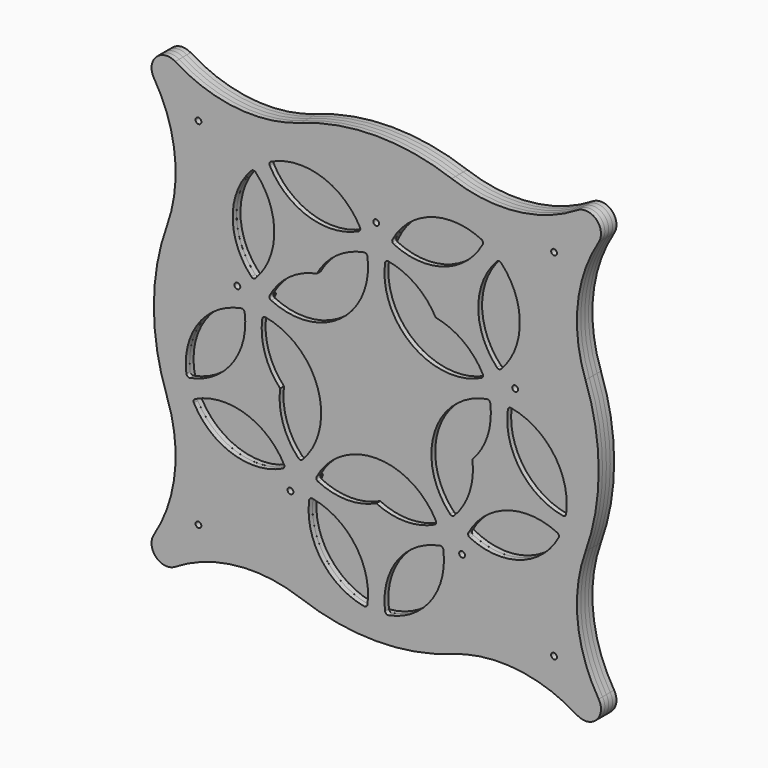
from build123d import *

# Parameters (mm, degrees)
F2_DEPTH  = 2.5
F4_DEPTH  = 2.5
F6_DEPTH  = 2.5
F8_DEPTH  = 2.5
F9_R      = 1.5
F10_DEPTH = 25
F11_DEPTH = 355


# Not quite as in the source:
# - an extrude ends at something that could not be found from the text; its depth is read off the source's solid


with BuildPart() as f2:
    # F1 (on Front) → F2 (new body)
    with BuildSketch(Plane.XZ):
        with BuildLine():
            ThreePointArc((24.0259388064, -87.5519624316), (57.2853373786, -83.5126697988), (88.9850116486, -94.3585966628))
            ThreePointArc((88.9850116486, -94.3585966628), (98.8568675438, -93.2159096685), (99.9995545382, -83.3440537732))
            ThreePointArc((99.9995545382, -83.3440537732), (89.1536276742, -51.6443795033), (93.192920307, -18.384980931))
            ThreePointArc((93.192920307, -18.384980931), (100.0126757728, 20.6282821025), (93.192920307, 59.6415451361))
            ThreePointArc((93.192920307, 59.6415451361), (89.1536276742, 92.9009437083), (99.9995545382, 124.6006179783))
            ThreePointArc((99.9995545382, 124.6006179783), (98.8568675438, 134.4724738736), (88.9850116486, 135.6151608679))
            ThreePointArc((88.9850116486, 135.6151608679), (57.2853373786, 124.7692340039), (24.0259388064, 128.8085266367))
            ThreePointArc((24.0259388064, 128.8085266367), (-14.9873242272, 135.6282821025), (-54.0005872607, 128.8085266367))
            ThreePointArc((-54.0005872607, 128.8085266367), (-87.259985833, 124.7692340039), (-118.959660103, 135.6151608679))
            ThreePointArc((-118.959660103, 135.6151608679), (-128.8315159982, 134.4724738736), (-129.9742029925, 124.6006179783))
            ThreePointArc((-129.9742029925, 124.6006179783), (-119.1282761286, 92.9009437083), (-123.1675687614, 59.6415451361))
            ThreePointArc((-123.1675687614, 59.6415451361), (-129.9873242272, 20.6282821025), (-123.1675687614, -18.384980931))
            ThreePointArc((-123.1675687614, -18.384980931), (-119.1282761286, -51.6443795033), (-129.9742029925, -83.3440537732))
            ThreePointArc((-129.9742029925, -83.3440537732), (-128.8315159982, -93.2159096685), (-118.959660103, -94.3585966628))
            ThreePointArc((-118.959660103, -94.3585966628), (-87.259985833, -83.5126697988), (-54.0005872607, -87.5519624316))
            ThreePointArc((-54.0005872607, -87.5519624316), (-14.9873242272, -94.3717178975), (24.0259388064, -87.5519624316))
        make_face()
        with BuildLine():
            ThreePointArc((-19.771685074, 80.7976974748), (-14.9873242272, 81.1262410403), (-10.2029633803, 80.7976974748))
            ThreePointArc((-10.2029633803, 80.7976974748), (44.8224838302, 102.9494205796), (40.7587415354, 43.7718515539))
            ThreePointArc((40.7587415354, 43.7718515539), (42.5496538431, 39.3231795393), (43.7156391532, 34.6714564345))
            ThreePointArc((43.7156391532, 34.6714564345), (81.7869780703, -10.8155948031), (24.25, -25.2376207278))
            ThreePointArc((24.25, -25.2376207278), (20.5724838302, -28.3155948031), (16.5087415354, -30.8619742226))
            ThreePointArc((16.5087415354, -30.8619742226), (-14.9873242272, -81.1262410403), (-46.4833899897, -30.8619742226))
            ThreePointArc((-46.4833899897, -30.8619742226), (-50.5471322846, -28.3155948031), (-54.2246484544, -25.2376207278))
            ThreePointArc((-54.2246484544, -25.2376207278), (-111.7616265247, -10.8155948031), (-73.6902876075, 34.6714564345))
            ThreePointArc((-73.6902876075, 34.6714564345), (-72.5243022975, 39.3231795393), (-70.7333899897, 43.7718515539))
            ThreePointArc((-70.7333899897, 43.7718515539), (-74.7971322846, 102.9494205796), (-19.771685074, 80.7976974748))
        make_face(mode=Mode.SUBTRACT)
        with BuildLine():
            ThreePointArc((40.7587415354, 43.7718515539), (44.8224838302, 102.9494205796), (-10.2029633803, 80.7976974748))
            ThreePointArc((-10.2029633803, 80.7976974748), (-14.9873242272, 81.1262410403), (-19.771685074, 80.7976974748))
            ThreePointArc((-19.771685074, 80.7976974748), (-74.7971322846, 102.9494205796), (-70.7333899897, 43.7718515539))
            ThreePointArc((-70.7333899897, 43.7718515539), (-72.5243022975, 39.3231795393), (-73.6902876075, 34.6714564345))
            ThreePointArc((-73.6902876075, 34.6714564345), (-111.7616265247, -10.8155948031), (-54.2246484544, -25.2376207278))
            ThreePointArc((-54.2246484544, -25.2376207278), (-50.5471322846, -28.3155948031), (-46.4833899897, -30.8619742226))
            ThreePointArc((-46.4833899897, -30.8619742226), (-14.9873242272, -81.1262410403), (16.5087415354, -30.8619742226))
            ThreePointArc((16.5087415354, -30.8619742226), (20.5724838302, -28.3155948031), (24.25, -25.2376207278))
            ThreePointArc((24.25, -25.2376207278), (81.7869780703, -10.8155948031), (43.7156391532, 34.6714564345))
            ThreePointArc((43.7156391532, 34.6714564345), (42.5496538431, 39.3231795393), (40.7587415354, 43.7718515539))
        make_face()
    extrude(amount=F2_DEPTH)


with BuildPart() as f4:
    # F3 (on face) → F4 (new body)
    with BuildSketch(Plane.XZ.offset(2.5)):
        with BuildLine():
            ThreePointArc((-54.0005872607, 128.8085266367), (-87.259985833, 124.7692340039), (-118.959660103, 135.6151608679))
            ThreePointArc((-118.959660103, 135.6151608679), (-128.8315159982, 134.4724738736), (-129.9742029925, 124.6006179783))
            ThreePointArc((-129.9742029925, 124.6006179783), (-119.1282761286, 92.9009437083), (-123.1675687614, 59.6415451361))
            ThreePointArc((-123.1675687614, 59.6415451361), (-129.9873242272, 20.6282821025), (-123.1675687614, -18.384980931))
            ThreePointArc((-123.1675687614, -18.384980931), (-119.1282761286, -51.6443795033), (-129.9742029925, -83.3440537732))
            ThreePointArc((-129.9742029925, -83.3440537732), (-128.8315159982, -93.2159096685), (-118.959660103, -94.3585966628))
            ThreePointArc((-118.959660103, -94.3585966628), (-87.259985833, -83.5126697988), (-54.0005872607, -87.5519624316))
            ThreePointArc((-54.0005872607, -87.5519624316), (-14.9873242272, -94.3717178975), (24.0259388064, -87.5519624316))
            ThreePointArc((24.0259388064, -87.5519624316), (57.2853373786, -83.5126697988), (88.9850116486, -94.3585966628))
            ThreePointArc((88.9850116486, -94.3585966628), (98.8568675438, -93.2159096685), (99.9995545382, -83.3440537732))
            ThreePointArc((99.9995545382, -83.3440537732), (89.1536276742, -51.6443795033), (93.192920307, -18.384980931))
            ThreePointArc((93.192920307, -18.384980931), (100.0126757728, 20.6282821025), (93.192920307, 59.6415451361))
            ThreePointArc((93.192920307, 59.6415451361), (89.1536276742, 92.9009437083), (99.9995545382, 124.6006179783))
            ThreePointArc((99.9995545382, 124.6006179783), (98.8568675438, 134.4724738736), (88.9850116486, 135.6151608679))
            ThreePointArc((88.9850116486, 135.6151608679), (57.2853373786, 124.7692340039), (24.0259388064, 128.8085266367))
            ThreePointArc((24.0259388064, 128.8085266367), (-14.9873242272, 135.6282821025), (-54.0005872607, 128.8085266367))
        make_face()
        with BuildLine():
            ThreePointArc((-51.5300809238, -32.5017435079), (-52.8982732938, -31.5516627806), (-54.2246484544, -30.5440256024))
            ThreePointArc((-54.2246484544, -30.5440256024), (-115.5658525899, -12.0516627806), (-76.8093141355, 38.9644281571))
            ThreePointArc((-76.8093141355, 38.9644281571), (-76.3285283627, 40.5592475168), (-75.7800809238, 42.1320822686))
            ThreePointArc((-75.7800809238, 42.1320822686), (-77.1482732938, 106.1854885571), (-16.652658546, 85.0906691974))
            ThreePointArc((-16.652658546, 85.0906691974), (-14.9873242272, 85.1262410403), (-13.3219899083, 85.0906691974))
            ThreePointArc((-13.3219899083, 85.0906691974), (47.1736248394, 106.1854885571), (45.8054324695, 42.1320822686))
            ThreePointArc((45.8054324695, 42.1320822686), (46.3538799083, 40.5592475168), (46.8346656811, 38.9644281571))
            ThreePointArc((46.8346656811, 38.9644281571), (85.5912041355, -12.0516627806), (24.25, -30.5440256024))
            ThreePointArc((24.25, -30.5440256024), (22.9236248394, -31.5516627806), (21.5554324695, -32.5017435079))
            ThreePointArc((21.5554324695, -32.5017435079), (-14.9873242272, -85.1262410403), (-51.5300809238, -32.5017435079))
        make_face(mode=Mode.SUBTRACT)
    extrude(amount=F4_DEPTH)


with BuildPart() as f6:
    # F5 (on face) → F6 (new body)
    with BuildSketch(Plane.XZ.offset(5)):
        with BuildLine():
            ThreePointArc((-129.9742029925, 124.6006179783), (-119.1282761286, 92.9009437083), (-123.1675687614, 59.6415451361))
            ThreePointArc((-123.1675687614, 59.6415451361), (-129.9873242272, 20.6282821025), (-123.1675687614, -18.384980931))
            ThreePointArc((-123.1675687614, -18.384980931), (-119.1282761286, -51.6443795033), (-129.9742029925, -83.3440537732))
            ThreePointArc((-129.9742029925, -83.3440537732), (-128.8315159982, -93.2159096685), (-118.959660103, -94.3585966628))
            ThreePointArc((-118.959660103, -94.3585966628), (-87.259985833, -83.5126697988), (-54.0005872607, -87.5519624316))
            ThreePointArc((-54.0005872607, -87.5519624316), (-14.9873242272, -94.3717178975), (24.0259388064, -87.5519624316))
            ThreePointArc((24.0259388064, -87.5519624316), (57.2853373786, -83.5126697988), (88.9850116486, -94.3585966628))
            ThreePointArc((88.9850116486, -94.3585966628), (98.8568675438, -93.2159096685), (99.9995545382, -83.3440537732))
            ThreePointArc((99.9995545382, -83.3440537732), (89.1536276742, -51.6443795033), (93.192920307, -18.384980931))
            ThreePointArc((93.192920307, -18.384980931), (100.0126757728, 20.6282821025), (93.192920307, 59.6415451361))
            ThreePointArc((93.192920307, 59.6415451361), (89.1536276742, 92.9009437083), (99.9995545382, 124.6006179783))
            ThreePointArc((99.9995545382, 124.6006179783), (98.8568675438, 134.4724738736), (88.9850116486, 135.6151608679))
            ThreePointArc((88.9850116486, 135.6151608679), (57.2853373786, 124.7692340039), (24.0259388064, 128.8085266367))
            ThreePointArc((24.0259388064, 128.8085266367), (-14.9873242272, 135.6282821025), (-54.0005872607, 128.8085266367))
            ThreePointArc((-54.0005872607, 128.8085266367), (-87.259985833, 124.7692340039), (-118.959660103, 135.6151608679))
            ThreePointArc((-118.959660103, 135.6151608679), (-128.8315159982, 134.4724738736), (-129.9742029925, 124.6006179783))
        make_face()
        with BuildLine():
            ThreePointArc((-73.6902876075, 34.6714564345), (-72.5243022975, 39.3231795393), (-70.7333899897, 43.7718515539))
            ThreePointArc((-70.7333899897, 43.7718515539), (-74.7971322846, 102.9494205796), (-19.771685074, 80.7976974748))
            ThreePointArc((-19.771685074, 80.7976974748), (-14.9873242272, 81.1262410403), (-10.2029633803, 80.7976974748))
            ThreePointArc((-10.2029633803, 80.7976974748), (44.8224838302, 102.9494205796), (40.7587415354, 43.7718515539))
            ThreePointArc((40.7587415354, 43.7718515539), (42.5496538431, 39.3231795393), (43.7156391532, 34.6714564345))
            ThreePointArc((43.7156391532, 34.6714564345), (81.7869780703, -10.8155948031), (24.25, -25.2376207278))
            ThreePointArc((24.25, -25.2376207278), (20.5724838302, -28.3155948031), (16.5087415354, -30.8619742226))
            ThreePointArc((16.5087415354, -30.8619742226), (-14.9873242272, -81.1262410403), (-46.4833899897, -30.8619742226))
            ThreePointArc((-46.4833899897, -30.8619742226), (-50.5471322846, -28.3155948031), (-54.2246484544, -25.2376207278))
            ThreePointArc((-54.2246484544, -25.2376207278), (-111.7616265247, -10.8155948031), (-73.6902876075, 34.6714564345))
        make_face(mode=Mode.SUBTRACT)
    extrude(amount=F6_DEPTH)


with BuildPart() as f8:
    # F7 (on face) → F8 (new body)
    with BuildSketch(Plane.XZ.offset(7.5)):
        with BuildLine():
            ThreePointArc((-129.9742029925, 124.6006179783), (-119.1282761286, 92.9009437083), (-123.1675687614, 59.6415451361))
            ThreePointArc((-123.1675687614, 59.6415451361), (-129.9873242272, 20.6282821025), (-123.1675687614, -18.384980931))
            ThreePointArc((-123.1675687614, -18.384980931), (-119.1282761286, -51.6443795033), (-129.9742029925, -83.3440537732))
            ThreePointArc((-129.9742029925, -83.3440537732), (-128.8315159982, -93.2159096685), (-118.959660103, -94.3585966628))
            ThreePointArc((-118.959660103, -94.3585966628), (-87.259985833, -83.5126697988), (-54.0005872607, -87.5519624316))
            ThreePointArc((-54.0005872607, -87.5519624316), (-14.9873242272, -94.3717178975), (24.0259388064, -87.5519624316))
            ThreePointArc((24.0259388064, -87.5519624316), (57.2853373786, -83.5126697988), (88.9850116486, -94.3585966628))
            ThreePointArc((88.9850116486, -94.3585966628), (98.8568675438, -93.2159096685), (99.9995545382, -83.3440537732))
            ThreePointArc((99.9995545382, -83.3440537732), (89.1536276742, -51.6443795033), (93.192920307, -18.384980931))
            ThreePointArc((93.192920307, -18.384980931), (100.0126757728, 20.6282821025), (93.192920307, 59.6415451361))
            ThreePointArc((93.192920307, 59.6415451361), (89.1536276742, 92.9009437083), (99.9995545382, 124.6006179783))
            ThreePointArc((99.9995545382, 124.6006179783), (98.8568675438, 134.4724738736), (88.9850116486, 135.6151608679))
            ThreePointArc((88.9850116486, 135.6151608679), (57.2853373786, 124.7692340039), (24.0259388064, 128.8085266367))
            ThreePointArc((24.0259388064, 128.8085266367), (-14.9873242272, 135.6282821025), (-54.0005872607, 128.8085266367))
            ThreePointArc((-54.0005872607, 128.8085266367), (-87.259985833, 124.7692340039), (-118.959660103, 135.6151608679))
            ThreePointArc((-118.959660103, 135.6151608679), (-128.8315159982, 134.4724738736), (-129.9742029925, 124.6006179783))
        make_face()
        with BuildLine():
            ThreePointArc((-49.6779104052, -41.4826184645), (-49.072848876, -40.468105369), (-47.9210152905, -40.2061594464))
            ThreePointArc((-47.9210152905, -40.2061594464), (-25.9090536512, -54.0613419463), (-19.5340622764, -79.2774483524))
            ThreePointArc((-19.5340622764, -79.2774483524), (-20.1391238056, -80.2919614478), (-21.290957391, -80.5539073704))
            ThreePointArc((-21.290957391, -80.5539073704), (-43.3029190303, -66.6987248706), (-49.6779104052, -41.4826184645))
        make_face(mode=Mode.SUBTRACT)
        with BuildLine():
            ThreePointArc((-109.2693750845, -16.6338453695), (-109.3761858605, -15.4574407906), (-108.5983008654, -14.568491293))
            ThreePointArc((-108.5983008654, -14.568491293), (-82.6463778784, -12.83926297), (-62.6672460514, -29.4923956708))
            ThreePointArc((-62.6672460514, -29.4923956708), (-62.5604352754, -30.6688002497), (-63.3383202706, -31.5577497473))
            ThreePointArc((-63.3383202706, -31.5577497473), (-89.2902432575, -33.2869780703), (-109.2693750845, -16.6338453695))
        make_face(mode=Mode.SUBTRACT)
        with BuildLine():
            ThreePointArc((-84.7782816182, 34.4276663301), (-83.6264480327, 34.1657204075), (-83.0213865036, 33.151207312))
            ThreePointArc((-83.0213865036, 33.151207312), (-89.3963778784, 7.9351009059), (-111.4083395177, -5.9200815939))
            ThreePointArc((-111.4083395177, -5.9200815939), (-112.5601731032, -5.6581356713), (-113.1652346324, -4.6436225759))
            ThreePointArc((-113.1652346324, -4.6436225759), (-106.7902432575, 20.5724838302), (-84.7782816182, 34.4276663301))
        make_face(mode=Mode.SUBTRACT)
        with BuildLine():
            ThreePointArc((15.8074024029, -29.4923956708), (15.914213179, -30.6688002497), (15.1363281838, -31.5577497473))
            ThreePointArc((15.1363281838, -31.5577497473), (0.0825353678, -34.9999026843), (-14.9873242272, -31.6287861371))
            ThreePointArc((-14.9873242272, -31.6287861371), (-30.0571838222, -34.9999026843), (-45.1109766382, -31.5577497473))
            ThreePointArc((-45.1109766382, -31.5577497473), (-45.8888616333, -30.6688002497), (-45.7820508573, -29.4923956708))
            ThreePointArc((-45.7820508573, -29.4923956708), (-14.9873242272, -11.1262410403), (15.8074024029, -29.4923956708))
        make_face(mode=Mode.SUBTRACT)
        with BuildLine():
            ThreePointArc((-53.1388275588, -24.1473845281), (-54.2246484544, -24.6124966198), (-55.3104693499, -24.1473845281))
            ThreePointArc((-55.3104693499, -24.1473845281), (-63.2360291407, -10.8940605303), (-64.686749499, 4.4799599403))
            ThreePointArc((-64.686749499, 4.4799599403), (-72.5497145761, 17.7705158047), (-73.9279104052, 33.151207312))
            ThreePointArc((-73.9279104052, 33.151207312), (-73.322848876, 34.1657204075), (-72.1710152905, 34.4276663301))
            ThreePointArc((-72.1710152905, 34.4276663301), (-45.187670384, 10.8155948031), (-53.1388275588, -24.1473845281))
        make_face(mode=Mode.SUBTRACT)
        with BuildLine():
            ThreePointArc((-8.6836910633, -80.5539073704), (-9.8355246488, -80.2919614478), (-10.440586178, -79.2774483524))
            ThreePointArc((-10.440586178, -79.2774483524), (-4.0655948031, -54.0613419463), (17.9463668362, -40.2061594464))
            ThreePointArc((17.9463668362, -40.2061594464), (19.0982004216, -40.468105369), (19.7032619508, -41.4826184645))
            ThreePointArc((19.7032619508, -41.4826184645), (13.3282705759, -66.6987248706), (-8.6836910633, -80.5539073704))
        make_face(mode=Mode.SUBTRACT)
        with BuildLine():
            ThreePointArc((34.7121010446, 4.4799599403), (33.2613806863, -10.8940605303), (25.3358208955, -24.1473845281))
            ThreePointArc((25.3358208955, -24.1473845281), (24.25, -24.6124966198), (23.1641791045, -24.1473845281))
            ThreePointArc((23.1641791045, -24.1473845281), (15.2130219297, 10.8155948031), (42.1963668362, 34.4276663301))
            ThreePointArc((42.1963668362, 34.4276663301), (43.3482004216, 34.1657204075), (43.9532619508, 33.151207312))
            ThreePointArc((43.9532619508, 33.151207312), (42.5750661217, 17.7705158047), (34.7121010446, 4.4799599403))
        make_face(mode=Mode.SUBTRACT)
        with BuildLine():
            ThreePointArc((79.2947266301, -16.6338453695), (59.3155948031, -33.2869780703), (33.3636718162, -31.5577497473))
            ThreePointArc((33.3636718162, -31.5577497473), (32.585786821, -30.6688002497), (32.6925975971, -29.4923956708))
            ThreePointArc((32.6925975971, -29.4923956708), (52.6717294241, -12.83926297), (78.623652411, -14.568491293))
            ThreePointArc((78.623652411, -14.568491293), (79.4015374061, -15.4574407906), (79.2947266301, -16.6338453695))
        make_face(mode=Mode.SUBTRACT)
        with BuildLine():
            ThreePointArc((83.190586178, -4.6436225759), (82.5855246488, -5.6581356713), (81.4336910633, -5.9200815939))
            ThreePointArc((81.4336910633, -5.9200815939), (59.4217294241, 7.9351009059), (53.0467380492, 33.151207312))
            ThreePointArc((53.0467380492, 33.151207312), (53.6517995784, 34.1657204075), (54.8036331638, 34.4276663301))
            ThreePointArc((54.8036331638, 34.4276663301), (76.8155948031, 20.5724838302), (83.190586178, -4.6436225759))
        make_face(mode=Mode.SUBTRACT)
        with BuildLine():
            ThreePointArc((-79.5604693499, 98.7812103046), (-78.4746484544, 99.2463223963), (-77.3888275588, 98.7812103046))
            ThreePointArc((-77.3888275588, 98.7812103046), (-67.7246484544, 74.6338257765), (-77.3888275588, 50.4864412484))
            ThreePointArc((-77.3888275588, 50.4864412484), (-78.4746484544, 50.0213291567), (-79.5604693499, 50.4864412484))
            ThreePointArc((-79.5604693499, 50.4864412484), (-89.2246484544, 74.6338257765), (-79.5604693499, 98.7812103046))
        make_face(mode=Mode.SUBTRACT)
        with BuildLine():
            ThreePointArc((-69.3609766382, 43.0760760292), (-70.1388616333, 43.9650255268), (-70.0320508573, 45.1414301057))
            ThreePointArc((-70.0320508573, 45.1414301057), (-59.8765233719, 56.7745877373), (-45.7032582665, 62.9051383847))
            ThreePointArc((-45.7032582665, 62.9051383847), (-35.4929783415, 74.4902701854), (-21.290957391, 80.5539073704))
            ThreePointArc((-21.290957391, 80.5539073704), (-20.1391238056, 80.2919614478), (-19.5340622764, 79.2774483524))
            ThreePointArc((-19.5340622764, 79.2774483524), (-33.6521646241, 46.3182309734), (-69.3609766382, 43.0760760292))
        make_face(mode=Mode.SUBTRACT)
        with BuildLine():
            ThreePointArc((-23.4299218242, 91.267671146), (-23.3231110482, 90.0912665671), (-24.1009960434, 89.2023170695))
            ThreePointArc((-24.1009960434, 89.2023170695), (-50.0529190303, 87.4730887465), (-70.0320508573, 104.1262214473))
            ThreePointArc((-70.0320508573, 104.1262214473), (-70.1388616333, 105.3026260262), (-69.3609766382, 106.1915755238))
            ThreePointArc((-69.3609766382, 106.1915755238), (-43.4090536512, 107.9208038468), (-23.4299218242, 91.267671146))
        make_face(mode=Mode.SUBTRACT)
        with BuildLine():
            ThreePointArc((-10.440586178, 79.2774483524), (-9.8355246488, 80.2919614478), (-8.6836910633, 80.5539073704))
            ThreePointArc((-8.6836910633, 80.5539073704), (5.5183298871, 74.4902701854), (15.7286098121, 62.9051383847))
            ThreePointArc((15.7286098121, 62.9051383847), (29.9018749176, 56.7745877373), (40.0574024029, 45.1414301057))
            ThreePointArc((40.0574024029, 45.1414301057), (40.164213179, 43.9650255268), (39.3863281838, 43.0760760292))
            ThreePointArc((39.3863281838, 43.0760760292), (3.6775161698, 46.3182309734), (-10.440586178, 79.2774483524))
        make_face(mode=Mode.SUBTRACT)
        with BuildLine():
            ThreePointArc((49.5858208955, 50.4864412484), (48.5, 50.0213291567), (47.4141791045, 50.4864412484))
            ThreePointArc((47.4141791045, 50.4864412484), (37.75, 74.6338257765), (47.4141791045, 98.7812103046))
            ThreePointArc((47.4141791045, 98.7812103046), (48.5, 99.2463223963), (49.5858208955, 98.7812103046))
            ThreePointArc((49.5858208955, 98.7812103046), (59.25, 74.6338257765), (49.5858208955, 50.4864412484))
        make_face(mode=Mode.SUBTRACT)
        with BuildLine():
            ThreePointArc((39.3863281838, 106.1915755238), (40.164213179, 105.3026260262), (40.0574024029, 104.1262214473))
            ThreePointArc((40.0574024029, 104.1262214473), (20.0782705759, 87.4730887465), (-5.873652411, 89.2023170695))
            ThreePointArc((-5.873652411, 89.2023170695), (-6.6515374061, 90.0912665671), (-6.5447266301, 91.267671146))
            ThreePointArc((-6.5447266301, 91.267671146), (13.4344051969, 107.9208038468), (39.3863281838, 106.1915755238))
        make_face(mode=Mode.SUBTRACT)
    extrude(amount=F8_DEPTH)


with BuildPart() as f10_tool:
    # F9 (on Front) → F10 (new body)
    with BuildSketch(Plane.XZ):
        with Locations((76.9365573271, -71.2955994517)):
            Circle(F9_R)
        with Locations((76.9365573271, 112.5521636568)):
            Circle(F9_R)
        with Locations((-106.9112057814, 112.5521636568)):
            Circle(F9_R)
        with Locations((-106.9112057814, -71.2955994517)):
            Circle(F9_R)
        with Locations((29.3904623209, -40.4525009728)):
            Circle(F9_R)
        with Locations((56.8174427531, 43.9590651778)):
            Circle(F9_R)
        with Locations((-14.9873242272, 96.1282821025)):
            Circle(F9_R)
        with Locations((-86.7920912075, 43.9590651778)):
            Circle(F9_R)
        with Locations((-59.3651107753, -40.4525009728)):
            Circle(F9_R)
    extrude(amount=F10_DEPTH)


with BuildPart() as f2_1:
    add(f2.part)

    # F10: cut by f10_tool
    add(f10_tool.part, mode=Mode.SUBTRACT)

    # F9 (on Front) → F11 (cut, through all)
    with BuildSketch(Plane.XZ):
        with Locations((76.9365573271, -71.2955994517)):
            Circle(F9_R)
        with Locations((76.9365573271, 112.5521636568)):
            Circle(F9_R)
        with Locations((-106.9112057814, 112.5521636568)):
            Circle(F9_R)
        with Locations((-106.9112057814, -71.2955994517)):
            Circle(F9_R)
        with Locations((29.3904623209, -40.4525009728)):
            Circle(F9_R)
        with Locations((56.8174427531, 43.9590651778)):
            Circle(F9_R)
        with Locations((-14.9873242272, 96.1282821025)):
            Circle(F9_R)
        with Locations((-86.7920912075, 43.9590651778)):
            Circle(F9_R)
        with Locations((-59.3651107753, -40.4525009728)):
            Circle(F9_R)
    extrude(amount=-F11_DEPTH, mode=Mode.SUBTRACT)


with BuildPart() as f4_1:
    add(f4.part)

    # F10: cut by f10_tool
    add(f10_tool.part, mode=Mode.SUBTRACT)


with BuildPart() as f6_1:
    add(f6.part)

    # F10: cut by f10_tool
    add(f10_tool.part, mode=Mode.SUBTRACT)


with BuildPart() as f8_1:
    add(f8.part)

    # F10: cut by f10_tool
    add(f10_tool.part, mode=Mode.SUBTRACT)


solid = Compound([f2_1.part, f4_1.part, f6_1.part, f8_1.part])
